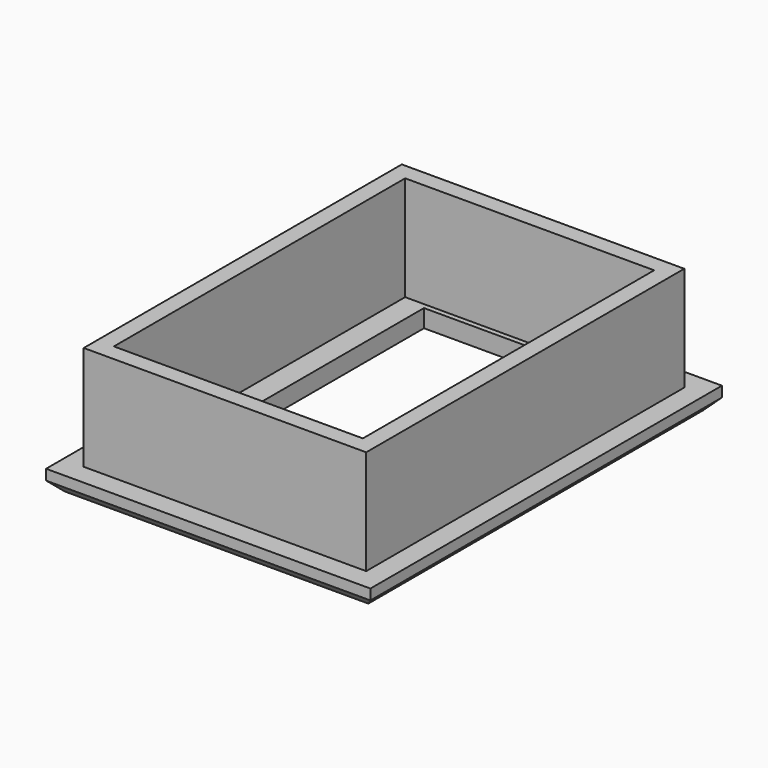
from build123d import *

# Parameters (mm, degrees)
F0_W     = 135
F0_H     = 190
F0_W_2   = 119
F0_H_2   = 174
F1_DEPTH = 50
F0_W_3   = 155
F0_H_3   = 210
F2_DEPTH = 10
F3_SIZE  = 5
F5_DEPTH = 1.5
F6_W     = 101.5
F6_H     = 170
F7_DEPTH = 60.001


# Not quite as in the source:
# - a feature names something its author has since deleted; it is built from what else it names


with BuildPart() as f1:
    # F0 (on Top) → F1 (new body)
    with BuildSketch(Plane.XY):
        with Locations((-101.2938845903, -16.7257675529)):
            Rectangle(F0_W, F0_H)
        with Locations((-101.2938845903, -16.7257675529)):
            Rectangle(F0_W_2, F0_H_2, mode=Mode.SUBTRACT)
    extrude(amount=F1_DEPTH)

    # F0 (on Top) → F2 (join)
    with BuildSketch(Plane.XY):
        with Locations((-101.2938845903, -16.7257675529)):
            Rectangle(F0_W_3, F0_H_3)
        with Locations((-101.2938845903, -16.7257675529)):
            Rectangle(F0_W, F0_H, mode=Mode.SUBTRACT)
        with Locations((-101.2938845903, -16.7257675529)):
            Rectangle(F0_W, F0_H)
        with Locations((-101.2938845903, -16.7257675529)):
            Rectangle(F0_W_2, F0_H_2, mode=Mode.SUBTRACT)
        with Locations((-101.2938845903, -16.7257675529)):
            Rectangle(F0_W_2, F0_H_2)
    extrude(amount=-F2_DEPTH)

    # F3
    f3_edges = [f1.edges().sort_by_distance(p)[0] for p in [
        (-101.293885, 88.274232, -10),
        (-178.793885, -16.725768, -10),
        (-101.293885, -121.725768, -10),
        (-23.793885, -16.725768, -10),
    ]]
    chamfer(f3_edges, length=F3_SIZE)

    # F4 (on face) → F5 (cut)
    with BuildSketch(Plane(origin=(0, 0, -10), x_dir=(1, 0, 0), z_dir=(0, 0, -1))):
        with BuildLine():
            Line((-53.2938845903, 113.2159726396), (-149.2938845903, 113.2159726396))
            ThreePointArc((-149.2938845903, 113.2159726396), (-154.5971854492, 111.0192734985), (-156.7938845903, 105.7159726396))
            Line((-156.7938845903, 105.7159726396), (-156.7938845903, -72.2840273604))
            ThreePointArc((-156.7938845903, -72.2840273604), (-154.5971854492, -77.5873282193), (-149.2938845903, -79.7840273604))
            Line((-149.2938845903, -79.7840273604), (-53.2938845903, -79.7840273604))
            ThreePointArc((-53.2938845903, -79.7840273604), (-47.9905837314, -77.5873282193), (-45.7938845903, -72.2840273604))
            Line((-45.7938845903, -72.2840273604), (-45.7938845903, 105.7159726396))
            ThreePointArc((-45.7938845903, 105.7159726396), (-47.9905837314, 111.0192734985), (-53.2938845903, 113.2159726396))
        make_face()
    extrude(amount=-F5_DEPTH, mode=Mode.SUBTRACT)

    # F6 (on face) → F7 (cut, through all)
    with BuildSketch(Plane(origin=(0, 0, -10), x_dir=(1, 0, 0), z_dir=(0, 0, -1))):
        with Locations((-99.0438845903, 17.2159726396)):
            Rectangle(F6_W, F6_H)
    extrude(amount=-F7_DEPTH, mode=Mode.SUBTRACT)


solid = f1.part
